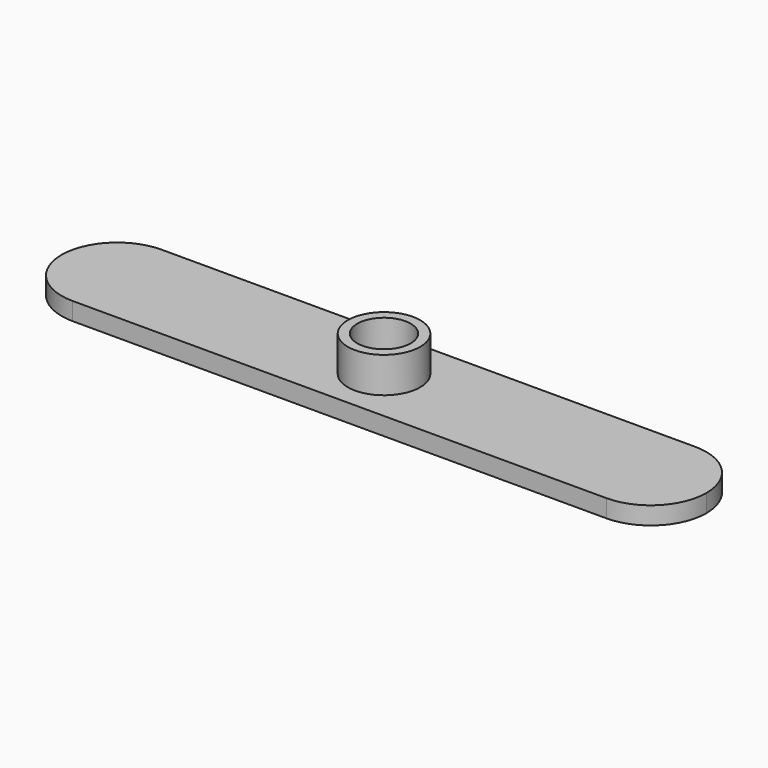
from build123d import *

# Parameters (mm, degrees)
F0_W     = 58
F0_H     = 10
F0_R     = 2.4
F1_DEPTH = 1.6
F2_R     = 3.255
F2_R_2   = 2.4
F3_DEPTH = 3.2
F4_R     = 4.99999


# Not quite as in the source:
# - a fillet or chamfer is up to 0.001 mm smaller than in the source, because OpenCascade refuses the exact size


with BuildPart() as f1:
    # F0 (on Top) → F1 (new body)
    with BuildSketch(Plane.XY):
        Rectangle(F0_W, F0_H)
        Circle(F0_R, mode=Mode.SUBTRACT)
    extrude(amount=-F1_DEPTH)

    # F2 (on face) → F3 (join)
    with BuildSketch(Plane.XY):
        Circle(F2_R)
        Circle(F2_R_2, mode=Mode.SUBTRACT)
    extrude(amount=F3_DEPTH)

    # F4 (radius 5 in the source; OpenCascade refuses exactly that, so slightly less here)
    f4_edges = [f1.edges().sort_by_distance(p)[0] for p in [
        (29, 5, -0.8),
        (29, -5, -0.8),
        (-29, 5, -0.8),
        (-29, -5, -0.8),
    ]]
    fillet(f4_edges, radius=F4_R)


solid = f1.part
